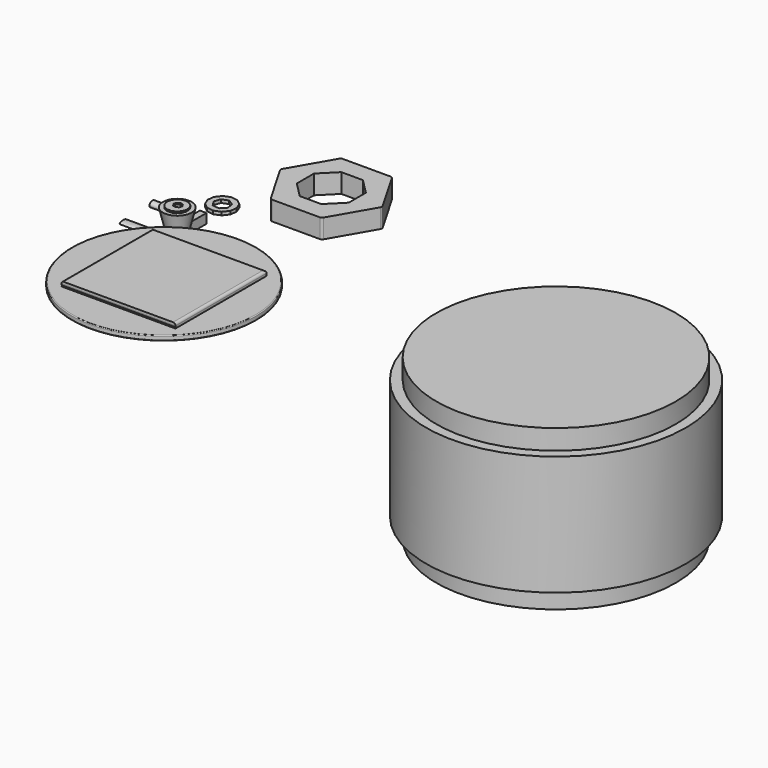
from build123d import *

# Parameters (mm, degrees)
F1_DEPTH  = 25.4
F3_DEPTH  = 51.308
F5_DEPTH  = 305.1048
F6_R      = 45.72
F7_R      = 1465.0405111475
F7_W      = 1814.1152858734
F7_H      = 1814.1152858734
F8_DEPTH  = 76.2
F9_DEPTH  = 76.2
F10_R     = 38.09999
F11_R     = 12.7
F12_R     = 1905
F13_DEPTH = 1270
F12_R_2   = 2063.75
F14_DEPTH = 952.5
F19_R     = 229.0809109199
F21_R     = 154.6394893279
F23_W     = 104.8123165965
F23_H     = 816.8393224478
F24_DEPTH = 76.2
F26_DEPTH = 643.5099393129


# Not quite as in the source:
# - a fillet or chamfer is up to 0.001 mm smaller than in the source, because OpenCascade refuses the exact size
# - the program builds the solid bodies; features that only make, move or delete a surface that nothing else refers to are left out


with BuildPart() as f1:
    # F0 (on Top) → F1 (new body)
    with BuildSketch(Plane.XY):
        Polygon((155.50936864, 47.9948012801), (122.5436329842, 107.0967912674), (68.3889899114, 147.6807731007), (2.4092691885, 162.7294076272), (-63.9870360646, 149.6406492247), (-119.3194014782, 110.6776631286), (-154.0203583934, 52.5775036026), (-162.0897961115, -14.6137839479), (-142.1324355422, -79.2782154918), (-97.5990856351, -130.2347233572), (-36.1899671618, -158.6724644088), (31.4767254093, -159.67429487), (93.7008062, -133.0669891528), (139.7231663537, -83.4511921354), (161.5861216997, -19.4059258675), align=None)
        Polygon((39.7706934855, 64.0896567419), (63.5851919651, 21.2782472372), (50.1523473576, -25.8333841012), (7.3409378529, -49.6478825808), (-39.7706934855, -36.2150379733), (-63.5851919651, 6.5963715315), (-50.1523473576, 53.7080028699), (-7.3409378529, 77.5225013494), align=None, mode=Mode.SUBTRACT)
    extrude(amount=F1_DEPTH)


with BuildPart() as f3:
    # F2 (on Top) → F3 (new body)
    with BuildSketch(Plane.XY):
        Polygon((567.1581641405, 172.1189159194), (635.2695226669, 258.6906254292), (650.9698346822, 367.7196043769), (610.052214261, 469.9916259019), (523.4805047512, 538.1029844284), (414.4515258035, 553.8032964437), (312.1795042784, 512.8856760224), (244.068145752, 426.3139665127), (228.3678337366, 317.284987565), (269.2854541579, 215.0129660399), (355.8571636677, 146.9016075134), (464.8861426154, 131.2012954981), align=None)
        Polygon((545.1443835194, 410.1638138472), (558.3316683769, 302.2244572639), (482.1634188256, 224.6151347452), (373.9958803268, 235.7772490893), (315.2814155857, 327.3055005294), (350.2332141092, 430.2772488952), (452.5318587224, 467.1526674262), align=None, mode=Mode.SUBTRACT)
    extrude(amount=F3_DEPTH)


with BuildPart() as f5:
    # F4 (on Top) → F5 (new body)
    with BuildSketch(Plane.XY):
        Polygon((1943.6769121667, 437.2407213386), (2349.1595144473, 1139.5571900737), (1943.6769121667, 1841.8736588088), (1132.7117076057, 1841.8736588088), (727.2291053252, 1139.5571900737), (1132.7117076057, 437.2407213386), align=None)
        Polygon((1709.2926557119, 1552.6251370658), (1951.2622568783, 1310.6555358994), (1951.2622568783, 968.458844248), (1709.2926557119, 726.4892430816), (1367.0959640605, 726.4892430816), (1125.1263628941, 968.458844248), (1125.1263628941, 1310.6555358994), (1367.0959640605, 1552.6251370658), align=None, mode=Mode.SUBTRACT)
    extrude(amount=F5_DEPTH)

    # F6
    f6_edges = [f5.edges().sort_by_distance(p)[0] for p in [
        (1943.676912, 437.240721, 152.5524),
        (2349.159514, 1139.55719, 152.5524),
        (1943.676912, 1841.873659, 152.5524),
        (1132.711708, 1841.873659, 152.5524),
        (727.229105, 1139.55719, 152.5524),
        (1132.711708, 437.240721, 152.5524),
    ]]
    fillet(f6_edges, radius=F6_R)


with BuildPart() as f8:
    # F7 (on Top) → F8 (new body)
    with BuildSketch(Plane.XY):
        with Locations((1112.9351854324, -1654.5432806015)):
            Circle(F7_R)
        with Locations((1112.9351854324, -1654.5432806015)):
            Rectangle(F7_W, F7_H, mode=Mode.SUBTRACT)
    extrude(amount=-F8_DEPTH)

    # F11
    f11_edges = [f8.edges().sort_by_distance(p)[0] for p in [
        (-352.105326, -1654.543281, 0),
        (-352.105326, -1654.543281, -76.2),
    ]]
    fillet(f11_edges, radius=F11_R)


with BuildPart() as f9:
    # F7 (on Top) → F9 (new body)
    with BuildSketch(Plane.XY):
        with Locations((1112.9351854324, -1654.5432806015)):
            Rectangle(F7_W, F7_H)
    extrude(amount=F9_DEPTH)

    # F10 (radius 38.1 in the source; OpenCascade refuses exactly that, so slightly less here)
    f10_edges = [f9.edges().sort_by_distance(p)[0] for p in [
        (205.877542, -1654.543281, 76.2),
        (2019.992828, -1654.543281, 76.2),
        (1112.935185, -2561.600924, 0),
        (1112.935185, -747.485638, 76.2),
    ]]
    fillet(f10_edges, radius=F10_R)


with BuildPart() as f13:
    # F12 (on Top) → F13 (new body, symmetric)
    with BuildSketch(Plane.XY):
        with Locations((7716.8588638306, -2116.8828010559)):
            Circle(F12_R)
    extrude(amount=F13_DEPTH, both=True)

    # F12 (on Top) → F14 (join, symmetric)
    with BuildSketch(Plane.XY):
        with Locations((7716.8588638306, -2116.8828010559)):
            Circle(F12_R_2)
        with Locations((7716.8588638306, -2116.8828010559)):
            Circle(F12_R, mode=Mode.SUBTRACT)
    extrude(amount=F14_DEPTH, both=True)


with BuildPart() as f22:
    # F19 (on Top) → F22 section 0
    with BuildSketch(Plane.XY):
        Circle(F19_R)
    # F21 (on offset) → F22 section 1
    with BuildSketch(Plane.XY.offset(-304.8)):
        Circle(F21_R)
    loft()

    # F23 (on offset) → F24 (join, symmetric)
    with BuildSketch(Plane.XY.offset(-304.8)):
        with Locations((52.4061582983, 40.6319275498)):
            Rectangle(F23_W, F23_H)
    extrude(amount=F24_DEPTH, both=True)

    # F25 (on face) → F26 (join)
    with BuildSketch(Plane(origin=(0, 0, 0), x_dir=(0, -1, 0), z_dir=(-1, 0, 0))):
        with BuildLine():
            add(Edge.make_bspline(
                [(204.6898007393, -302.1550476551), (204.6898007393, -345.0046976312), (306.7133426666, -323.5798726431), (408.736884594, -302.1550476551), (306.7133426666, -280.7302226671), (204.6898007393, -259.305397679), (204.6898007393, -302.1550476551)],
                knots=[0, 0, 0, 2.0943951024, 2.0943951024, 4.1887902048, 4.1887902048, 6.2831853072, 6.2831853072, 6.2831853072], degree=2, weights=[1, 0.5, 1, 0.5, 1, 0.5, 1]))
        make_face()
        with BuildLine():
            add(Edge.make_bspline(
                [(-369.6652650833, -287.2584462166), (-369.6652650833, -367.9612465382), (-280.7216048241, -327.6098463774), (-191.7779445648, -287.2584462166), (-280.7216048241, -246.9070460558), (-369.6652650833, -206.555645895), (-369.6652650833, -287.2584462166)],
                knots=[0, 0, 0, 2.0943951024, 2.0943951024, 4.1887902048, 4.1887902048, 6.2831853072, 6.2831853072, 6.2831853072], degree=2, weights=[1, 0.5, 1, 0.5, 1, 0.5, 1]))
        make_face()
    extrude(amount=F26_DEPTH)


solid = Compound([f1.part, f3.part, f5.part, f8.part, f9.part, f13.part, f22.part])
